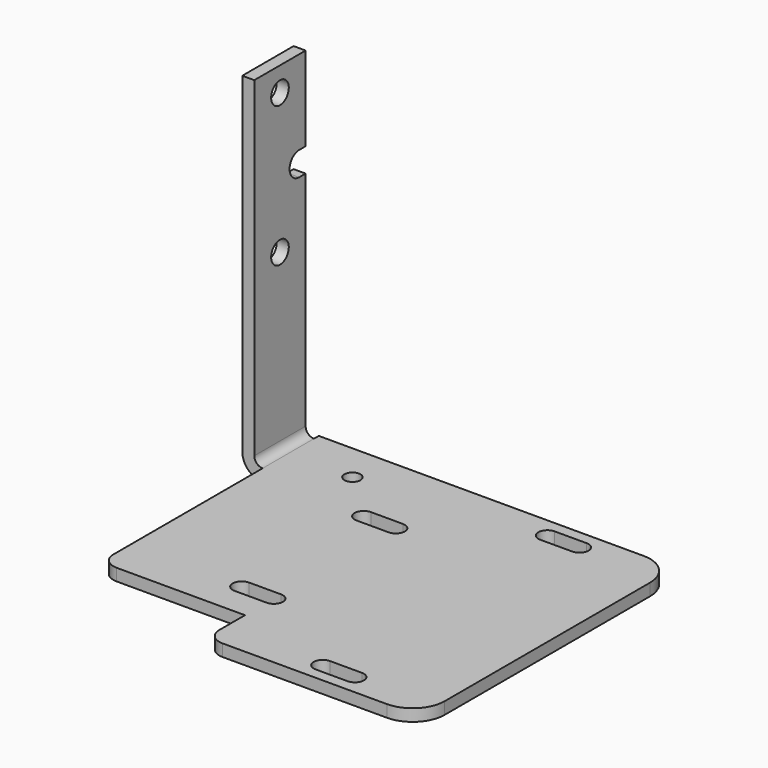
from build123d import *

# Parameters (mm, degrees)
F1_DEPTH = 127
F2_W     = 8.0518
F2_H     = 2.3876
F2_H_2   = 99.2124
F3_DEPTH = 138.90725
F5_DEPTH = 4.7635
F6_R     = 4.365625
F7_DEPTH = 149.3403


# Not quite as in the source:
# - a feature names something its author has since deleted; it is built from what else it names


with BuildPart() as f1:
    # F0 (on Front) → F1 (new body)
    with BuildSketch(Plane.XZ):
        with BuildLine():
            ThreePointArc((-8.0518, 8.0518), (-5.6934823808, 2.3583176192), (0, 0))
            Line((0, 0), (141.2875, 0))
            Line((141.2875, 0), (141.2875, 4.7625))
            Line((141.2875, 4.7625), (0, 4.7625))
            ThreePointArc((0, 4.7625), (-2.3258863354, 5.7259136646), (-3.2893, 8.0518))
            Line((-3.2893, 8.0518), (-3.2893, 138.90625))
            Line((-3.2893, 138.90625), (-8.0518, 138.90625))
            Line((-8.0518, 138.90625), (-8.0518, 8.0518))
        make_face()
    extrude(amount=-F1_DEPTH)

    # F2 (on face) → F3 (cut, through all)
    with BuildSketch(Plane.XY.offset(138.90625)):
        with Locations((-4.0259, 125.8062)):
            Rectangle(F2_W, F2_H)
        with Locations((-4.0259, 49.6062)):
            Rectangle(F2_W, F2_H_2)
    extrude(amount=-F3_DEPTH, mode=Mode.SUBTRACT)

    # F4 (on face) → F5 (cut, through all)
    with BuildSketch(Plane.XY.offset(4.7625)):
        with BuildLine():
            Line((44.45, 90.090625), (57.15, 90.090625))
            ThreePointArc((57.15, 90.090625), (60.721875, 93.6625), (57.15, 97.234375))
            Line((57.15, 97.234375), (44.45, 97.234375))
            ThreePointArc((44.45, 97.234375), (40.878125, 93.6625), (44.45, 90.090625))
        make_face()
        with BuildLine():
            Line((96.8380470509, 115.4906250419), (109.5212624401, 115.490625))
            ThreePointArc((109.5212624401, 115.490625), (113.0931374401, 119.0625055472), (109.5212513457, 122.634375))
            Line((109.5212513457, 122.634375), (96.8212513457, 122.6343355532))
            ThreePointArc((96.8212513457, 122.6343355532), (93.2493862179, 119.0540626774), (96.8380470509, 115.4906250419))
        make_face()
        with BuildLine():
            Line((44.4505470509, 29.7656250419), (57.0326853587, 29.7675520605))
            Line((57.0326853587, 29.7675520605), (57.2684081472, 29.7675881627))
            ThreePointArc((57.2684081472, 29.7675881627), (60.7213841756, 33.3967122102), (57.15, 36.909375))
            Line((57.15, 36.909375), (44.45, 36.909375))
            ThreePointArc((44.45, 36.909375), (40.8781250105, 33.3372264746), (44.4505470509, 29.7656250419))
        make_face()
        with BuildLine():
            Line((141.2875, 127), (128.5875, 127))
            ThreePointArc((128.5875, 127), (137.5677561211, 123.2802561211), (141.2875, 114.3))
            Line((141.2875, 114.3), (141.2875, 127))
        make_face()
        with BuildLine():
            ThreePointArc((6.35, 19.05), (1.8598719395, 20.9098719395), (0, 25.4))
            Line((0, 25.4), (0, 0))
            Line((0, 0), (63.5, 0))
            ThreePointArc((63.5, 0), (59.0098719395, 1.8598719395), (57.15, 6.35))
            Line((57.15, 6.35), (57.15, 19.05))
            Line((57.15, 19.05), (6.35, 19.05))
        make_face()
        with BuildLine():
            ThreePointArc((28.575, 111.9124), (25.4, 115.0874), (22.225, 111.9124))
            ThreePointArc((22.225, 111.9124), (25.4, 108.7374), (28.575, 111.9124))
        make_face()
        with BuildLine():
            Line((96.8380470509, 4.3656250419), (109.5212624401, 4.365625))
            ThreePointArc((109.5212624401, 4.365625), (113.0931374401, 7.9375055472), (109.5212513457, 11.509375))
            Line((109.5212513457, 11.509375), (96.8212513457, 11.5093355532))
            ThreePointArc((96.8212513457, 11.5093355532), (93.2493862179, 7.9290626774), (96.8380470509, 4.3656250419))
        make_face()
        with BuildLine():
            Line((141.2875, 0), (141.2875, 12.7))
            ThreePointArc((141.2875, 12.7), (137.5677561211, 3.7197438789), (128.5875, 0))
            Line((128.5875, 0), (141.2875, 0))
        make_face()
    extrude(amount=-F5_DEPTH, mode=Mode.SUBTRACT)

    # F6 (on face) → F7 (cut, through all)
    with BuildSketch(Plane(origin=(-8.0518, 0, 0), x_dir=(0, -1, 0), z_dir=(-1, 0, 0))):
        with BuildLine():
            Line((-121.4374, 105.56875), (-124.6124, 105.56875))
            Line((-124.6124, 105.56875), (-124.6124, 96.0440792053))
            Line((-124.6124, 96.0440792053), (-121.4933961759, 96.0440792053))
            Line((-121.4933961759, 96.0440792053), (-121.3814038241, 96.0440792053))
            ThreePointArc((-121.3814038241, 96.0440792053), (-116.674982302, 100.8342485718), (-121.4374, 105.56875))
        make_face()
        with Locations((-111.9124, 129.38125)):
            Circle(F6_R)
        with Locations((-111.9124, 73.81875)):
            Circle(F6_R)
    extrude(amount=-F7_DEPTH, mode=Mode.SUBTRACT)


solid = f1.part
